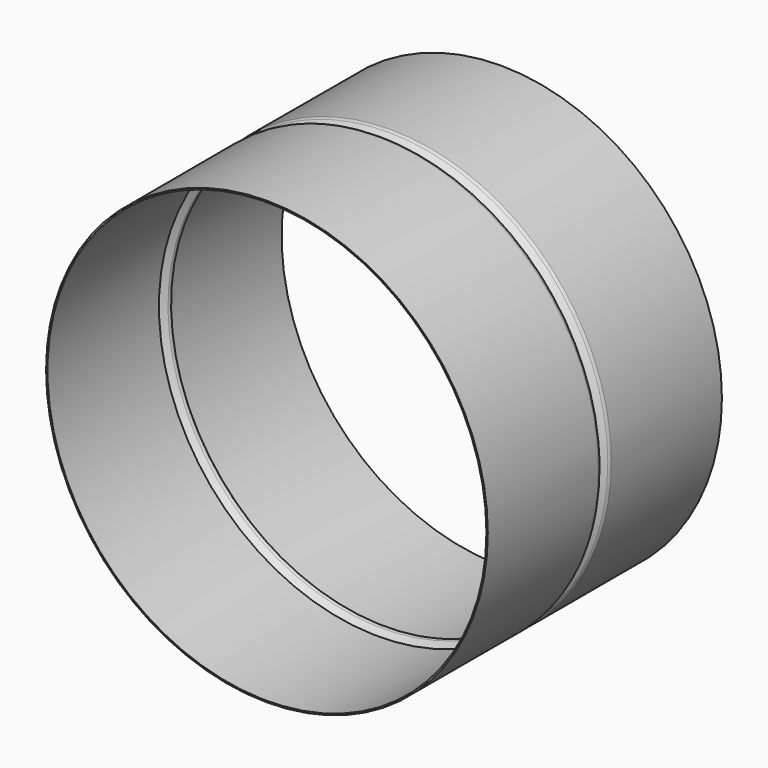
from build123d import *

# Parameters (mm, degrees)
F0_R     = 157.5
F1_DEPTH = 100
F2_R     = 157.5
F3_DEPTH = 5
F3_TAPER = 45
F4_T     = 1
F6_R     = 2
F7_R     = 3


with BuildPart() as f1:
    # F0 (on Front) → F1 (new body)
    with BuildSketch(Plane.XZ):
        Circle(F0_R)
    extrude(amount=F1_DEPTH)

    # F2 (on face) → F3 (join)
    with BuildSketch(Plane.XZ.offset(100)):
        Circle(F2_R)
    extrude(amount=F3_DEPTH, taper=F3_TAPER)

    # F4
    f4_openings = [f1.faces().sort_by_distance(p)[0] for p in [
        (0, -105, 0),
        (0, 0, 0),
    ]]
    offset(amount=F4_T, openings=f4_openings, kind=Kind.INTERSECTION)

    # F5: F1 across face


with BuildPart() as f1_1:
    add(f1.part)
    add(f1.part.mirror(Plane.XZ.offset(105)))

    # F6
    f6_edges = [f1_1.edges().sort_by_distance(p)[0] for p in [
        (-152.5, -105, 0),
    ]]
    fillet(f6_edges, radius=F6_R)

    # F7
    f7_edges = [f1_1.edges().sort_by_distance(p)[0] for p in [
        (-158.5, -100.414214, 0),
        (-158.5, -109.585786, 0),
    ]]
    fillet(f7_edges, radius=F7_R)


solid = f1_1.part
